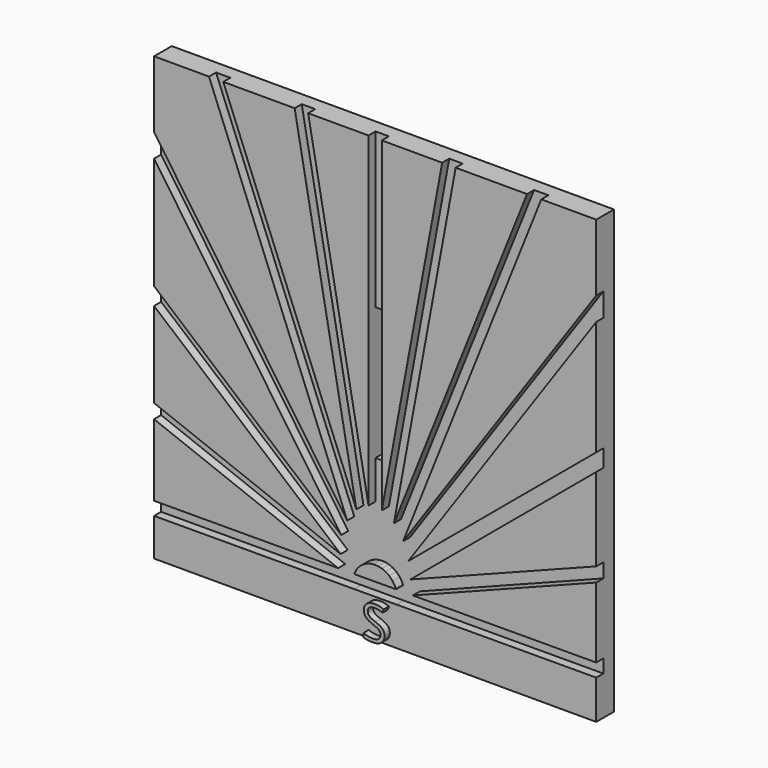
from build123d import *

# Parameters (mm, degrees)
F0_W          = 100
F0_H          = 100
F0_W_2        = 3
F0_H_2        = 30
F1_DEPTH      = 5
F3_DEPTH      = 2
F5_DEPTH      = 2
F7_DEPTH      = 2
F9_DEPTH      = 2
F11_DEPTH     = 2
F12_W         = 1.5
F12_H         = 35
F13_DEPTH     = 2
F15_DEPTH     = 2
F17_DEPTH     = 2
F19_DEPTH     = 2
F21_DEPTH     = 2
F23_DEPTH     = 2
F25_DEPTH     = 2
F26_TEXT_SIZE = 10.6048053024
F27_DEPTH     = 1.5


# Not quite as in the source:
# - a feature names something its author has since deleted; it is built from what else it names
# - Text() gives the source's letters only with a copy of the font that has no kerning and outlines rounded to 1/6400 em; it was checked with that copy


with BuildPart() as f1:
    # F0 (on Front) → F1 (new body)
    with BuildSketch(Plane.XZ):
        Rectangle(F0_W, F0_H)
        Rectangle(F0_W_2, F0_H_2, mode=Mode.SUBTRACT)
    extrude(amount=F1_DEPTH)

    # F2 (on face) → F3 (cut)
    with BuildSketch(Plane.XZ.offset(5)):
        with BuildLine():
            Line((-50, -20.6363906269), (-4.6625650979, -38.1943182153))
            ThreePointArc((-4.6625650979, -38.1943182153), (-4.3345358773, -37.5076519648), (-3.9060990907, -36.8787198309))
            Line((-3.9060990907, -36.8787198309), (-50, -19.0278339971))
            Line((-50, -19.0278339971), (-50, -20.6363906269))
        make_face()
        with BuildLine():
            ThreePointArc((-4.9895081615, -39.6762588897), (-4.8825881039, -38.9228122689), (-4.6625650979, -38.1943182153))
            Line((-4.6625650979, -38.1943182153), (-50, -20.6363906269))
            Line((-50, -20.6363906269), (-50, -22.2449472567))
            Line((-50, -22.2449472567), (-4.9895081615, -39.6762588897))
        make_face()
    extrude(amount=-F3_DEPTH, mode=Mode.SUBTRACT)

    # F4 (on face) → F5 (cut)
    with BuildSketch(Plane.XZ.offset(5)):
        with BuildLine():
            ThreePointArc((-3.8183618976, -36.7719801086), (-3.2842597112, -36.2299021035), (-2.6740791319, -35.7751567134))
            Line((-2.6740791319, -35.7751567134), (-50, 4.2338885364))
            Line((-50, 4.2338885364), (-50, 2.2696954607))
            Line((-50, 2.2696954607), (-3.8183618976, -36.7719801086))
        make_face()
        with BuildLine():
            ThreePointArc((-3.9060990907, -36.8787198309), (-3.8625992197, -36.8250468873), (-3.8183618976, -36.7719801086))
            Line((-3.8183618976, -36.7719801086), (-50, 2.2696954607))
            Line((-50, 2.2696954607), (-50, 0.3055023849))
            Line((-50, 0.3055023849), (-7.7986909066, -35.3712272835))
            Line((-7.7986909066, -35.3712272835), (-3.9060990907, -36.8787198309))
        make_face()
    extrude(amount=-F5_DEPTH, mode=Mode.SUBTRACT)

    # F6 (on face) → F7 (cut)
    with BuildSketch(Plane.XZ.offset(5)):
        with BuildLine():
            ThreePointArc((-2.6740791319, -35.7751567134), (-2.0954310446, -35.4602677681), (-1.4804072251, -35.2241865145))
            Line((-1.4804072251, -35.2241865145), (-50, 34.8992910693))
            Line((-50, 34.8992910693), (-50, 32.2630524839))
            Line((-50, 32.2630524839), (-3.2743801807, -35.267665863))
            Line((-3.2743801807, -35.267665863), (-2.6740791319, -35.7751567134))
        make_face()
        Polygon((-7.6690842868, -31.5524097789), (-3.2743801807, -35.267665863), (-50, 32.2630524839), (-50, 29.6268138986), align=None)
    extrude(amount=-F7_DEPTH, mode=Mode.SUBTRACT)

    # F8 (on face) → F9 (cut)
    with BuildSketch(Plane.XZ.offset(5)):
        Polygon((-2.4930135549, -33.7607060274), (-35.9609950948, 50), (-37.5763032154, 50), (-6.3160295281, -28.2354499491), align=None)
        with BuildLine():
            Line((-34.3456869742, 50), (-35.9609950948, 50))
            Line((-35.9609950948, 50), (-2.4930135549, -33.7607060274))
            Line((-2.4930135549, -33.7607060274), (-1.4804072251, -35.2241865145))
            ThreePointArc((-1.4804072251, -35.2241865145), (-0.9345403043, -35.0881129472), (-0.3768426, -35.0142212589))
            Line((-0.3768426, -35.0142212589), (-34.3456869742, 50))
        make_face()
    extrude(amount=-F9_DEPTH, mode=Mode.SUBTRACT)

    # F10 (on face) → F11 (cut)
    with BuildSketch(Plane.XZ.offset(5)):
        Polygon((-4.242855776, -25.3387051914), (-1.3974843117, -32.4598493953), (-16.6805140438, 50), (-18.2060594426, 50), align=None)
        with BuildLine():
            ThreePointArc((-0.3768426, -35.0142212589), (0.1149724294, -35.0013220407), (0.6056743031, -35.0368197052))
            Line((0.6056743031, -35.0368197052), (-15.1549686451, 50))
            Line((-15.1549686451, 50), (-16.6805140438, 50))
            Line((-16.6805140438, 50), (-1.3974843117, -32.4598493953))
            Line((-1.3974843117, -32.4598493953), (-0.3768426, -35.0142212589))
        make_face()
    extrude(amount=-F11_DEPTH, mode=Mode.SUBTRACT)

    # F12 (on face) → F13 (cut)
    with BuildSketch(Plane.XZ.offset(5)):
        with Locations((-0.75, 32.5)):
            Rectangle(F12_W, F12_H)
        with Locations((0.75, 32.5)):
            Rectangle(F12_W, F12_H)
        Polygon((0, -31.768893601), (0, -15), (-1.5, -15), (-1.5, -23.6756178395), align=None)
        with BuildLine():
            Line((1.5, -15), (0, -15))
            Line((0, -15), (0, -31.768893601))
            Line((0, -31.768893601), (0.6056743031, -35.0368197052))
            ThreePointArc((0.6056743031, -35.0368197052), (1.0572724862, -35.1130607851), (1.5, -35.2303039929))
            Line((1.5, -35.2303039929), (1.5, -15))
        make_face()
        with BuildLine():
            Line((0, -35), (0, -31.768893601))
            Line((0, -31.768893601), (-1.5, -23.6756178395))
            Line((-1.5, -23.6756178395), (-1.5, -35.2303039929))
            ThreePointArc((-1.5, -35.2303039929), (-0.7587884964, -35.0579113709), (0, -35))
        make_face()
    extrude(amount=-F13_DEPTH, mode=Mode.SUBTRACT)

    # F14 (on face) → F15 (cut)
    with BuildSketch(Plane.XZ.offset(5)):
        with BuildLine():
            ThreePointArc((1.5, -35.2303039929), (1.9301422965, -35.3875656411), (2.3440904196, -35.5835262817))
            Line((2.3440904196, -35.5835262817), (18.2060594426, 50))
            Line((18.2060594426, 50), (16.6805140438, 50))
            Line((16.6805140438, 50), (1.5, -31.9067242385))
            Line((1.5, -31.9067242385), (1.5, -35.2303039929))
        make_face()
        Polygon((1.5, -23.6756178395), (1.5, -31.9067242385), (16.6805140438, 50), (15.1549686451, 50), align=None)
    extrude(amount=-F15_DEPTH, mode=Mode.SUBTRACT)

    # F16 (on face) → F17 (cut)
    with BuildSketch(Plane.XZ.offset(5)):
        Polygon((4.242855776, -25.3387051914), (2.8453714643, -32.8788557961), (35.9609950948, 50), (34.3456869742, 50), align=None)
        with BuildLine():
            ThreePointArc((2.3440904196, -35.5835262817), (2.7667835242, -35.8352780489), (3.1626888064, -36.1273523896))
            Line((3.1626888064, -36.1273523896), (37.5763032154, 50))
            Line((37.5763032154, 50), (35.9609950948, 50))
            Line((35.9609950948, 50), (2.8453714643, -32.8788557961))
            Line((2.8453714643, -32.8788557961), (2.3440904196, -35.5835262817))
        make_face()
    extrude(amount=-F17_DEPTH, mode=Mode.SUBTRACT)

    # F18 (on face) → F19 (cut)
    with BuildSketch(Plane.XZ.offset(5)):
        Polygon((3.8230159732, -34.4747439217), (50, 32.2630524839), (50, 34.8992910693), (6.3160295281, -28.2354499491), align=None)
        with BuildLine():
            Line((50, 29.6268138986), (50, 32.2630524839))
            Line((50, 32.2630524839), (3.8230159732, -34.4747439217))
            Line((3.8230159732, -34.4747439217), (3.1626888064, -36.1273523896))
            ThreePointArc((3.1626888064, -36.1273523896), (3.5777080171, -36.5071493956), (3.947435346, -36.9311640336))
            Line((3.947435346, -36.9311640336), (50, 29.6268138986))
        make_face()
    extrude(amount=-F19_DEPTH, mode=Mode.SUBTRACT)

    # F20 (on face) → F21 (cut)
    with BuildSketch(Plane.XZ.offset(5)):
        Polygon((4.3152720076, -36.3995440339), (50, 1.7176015751), (50, 3.6711425788), (7.5130329599, -31.7779446835), align=None)
        with BuildLine():
            Line((50, -0.2359394286), (50, 1.7176015751))
            Line((50, 1.7176015751), (4.3152720076, -36.3995440339))
            Line((4.3152720076, -36.3995440339), (3.947435346, -36.9311640336))
            ThreePointArc((3.947435346, -36.9311640336), (4.3247765716, -37.4907555707), (4.6233153358, -38.0960684609))
            Line((4.6233153358, -38.0960684609), (50, -0.2359394286))
        make_face()
    extrude(amount=-F21_DEPTH, mode=Mode.SUBTRACT)

    # F22 (on face) → F23 (cut)
    with BuildSketch(Plane.XZ.offset(5)):
        with BuildLine():
            Line((50, -22.2449472567), (50, -20.6363906269))
            Line((50, -20.6363906269), (4.6625650979, -38.1943182153))
            ThreePointArc((4.6625650979, -38.1943182153), (4.8825881039, -38.9228122689), (4.9895081615, -39.6762588897))
            Line((4.9895081615, -39.6762588897), (50, -22.2449472567))
        make_face()
        with BuildLine():
            Line((4.6625650979, -38.1943182153), (50, -20.6363906269))
            Line((50, -20.6363906269), (50, -19.0278339971))
            Line((50, -19.0278339971), (7.9674753423, -35.3058617659))
            Line((7.9674753423, -35.3058617659), (4.6233153358, -38.0960684609))
            ThreePointArc((4.6233153358, -38.0960684609), (4.6432000938, -38.14508952), (4.6625650979, -38.1943182153))
        make_face()
    extrude(amount=-F23_DEPTH, mode=Mode.SUBTRACT)

    # F24 (on face) → F25 (cut)
    with BuildSketch(Plane.XZ.offset(5)):
        with BuildLine():
            Line((-50, -40), (-4.9978769808, -39.8543096273))
            ThreePointArc((-4.9978769808, -39.8543096273), (-4.9944860608, -39.7652469625), (-4.9895081615, -39.6762588897))
            Line((-4.9895081615, -39.6762588897), (-8.3747878606, -38.3652342155))
            Line((-8.3747878606, -38.3652342155), (-50, -38.4999921394))
            Line((-50, -38.4999921394), (-50, -40))
        make_face()
        with BuildLine():
            ThreePointArc((-4.8132569754, -41.353719797), (-4.9625240645, -40.6110277482), (-4.9978769808, -39.8543096273))
            Line((-4.9978769808, -39.8543096273), (-50, -40))
            Line((-50, -40), (-50, -41.5000078606))
            Line((-50, -41.5000078606), (-4.8132569754, -41.353719797))
        make_face()
        with BuildLine():
            Line((-4.9978769808, -39.8543096273), (4.9968289087, -39.8219526555))
            ThreePointArc((4.9968289087, -39.8219526555), (4.9936998997, -39.7490790728), (4.9895081615, -39.6762588897))
            ThreePointArc((4.9895081615, -39.6762588897), (4.8969017134, -38.9898744586), (4.7103336051, -38.3228722979))
            Line((4.7103336051, -38.3228722979), (-4.7210938596, -38.3534057059))
            ThreePointArc((-4.7210938596, -38.3534057059), (-4.9001462263, -39.005732953), (-4.9895081615, -39.6762588897))
            ThreePointArc((-4.9895081615, -39.6762588897), (-4.9944860608, -39.7652469625), (-4.9978769808, -39.8543096273))
        make_face()
        with BuildLine():
            ThreePointArc((4.8219210857, -41.3225267646), (4.9552802861, -40.6672310587), (5, -40))
            ThreePointArc((5, -40), (4.9992071643, -39.9109622093), (4.9968289087, -39.8219526555))
            Line((4.9968289087, -39.8219526555), (-4.9978769808, -39.8543096273))
            ThreePointArc((-4.9978769808, -39.8543096273), (-4.9625240645, -40.6110277482), (-4.8132569754, -41.353719797))
            Line((-4.8132569754, -41.353719797), (4.8219210857, -41.3225267646))
        make_face()
        with BuildLine():
            ThreePointArc((4.9895081615, -39.6762588897), (4.9936998997, -39.7490790728), (4.9968289087, -39.8219526555))
            Line((4.9968289087, -39.8219526555), (50, -39.6762588897))
            Line((50, -39.6762588897), (50, -38.1762510291))
            Line((50, -38.1762510291), (8.515986694, -38.3105518344))
            Line((8.515986694, -38.3105518344), (4.9895081615, -39.6762588897))
        make_face()
        with BuildLine():
            ThreePointArc((4.9968289087, -39.8219526555), (4.9992071643, -39.9109622093), (5, -40))
            ThreePointArc((5, -40), (4.9552802861, -40.6672310587), (4.8219210857, -41.3225267646))
            Line((4.8219210857, -41.3225267646), (50, -41.1762667503))
            Line((50, -41.1762667503), (50, -39.6762588897))
            Line((50, -39.6762588897), (4.9968289087, -39.8219526555))
        make_face()
        with BuildLine():
            Line((-8.3747878606, -38.3652342155), (-4.9895081615, -39.6762588897))
            ThreePointArc((-4.9895081615, -39.6762588897), (-4.9001462263, -39.005732953), (-4.7210938596, -38.3534057059))
            Line((-4.7210938596, -38.3534057059), (-8.3747878606, -38.3652342155))
        make_face()
        with BuildLine():
            ThreePointArc((4.7103336051, -38.3228722979), (4.8969017134, -38.9898744586), (4.9895081615, -39.6762588897))
            Line((4.9895081615, -39.6762588897), (8.515986694, -38.3105518344))
            Line((8.515986694, -38.3105518344), (4.7103336051, -38.3228722979))
        make_face()
    extrude(amount=-F25_DEPTH, mode=Mode.SUBTRACT)

    # F26 (on face) → F27 (join)
    with BuildSketch(Plane.XZ.offset(5)):
        with Locations((-2, -49.5)):
            Text('S', F26_TEXT_SIZE, font='Open Sans', text_align=(TextAlign.LEFT, TextAlign.BOTTOM))
    extrude(amount=F27_DEPTH)


solid = f1.part
